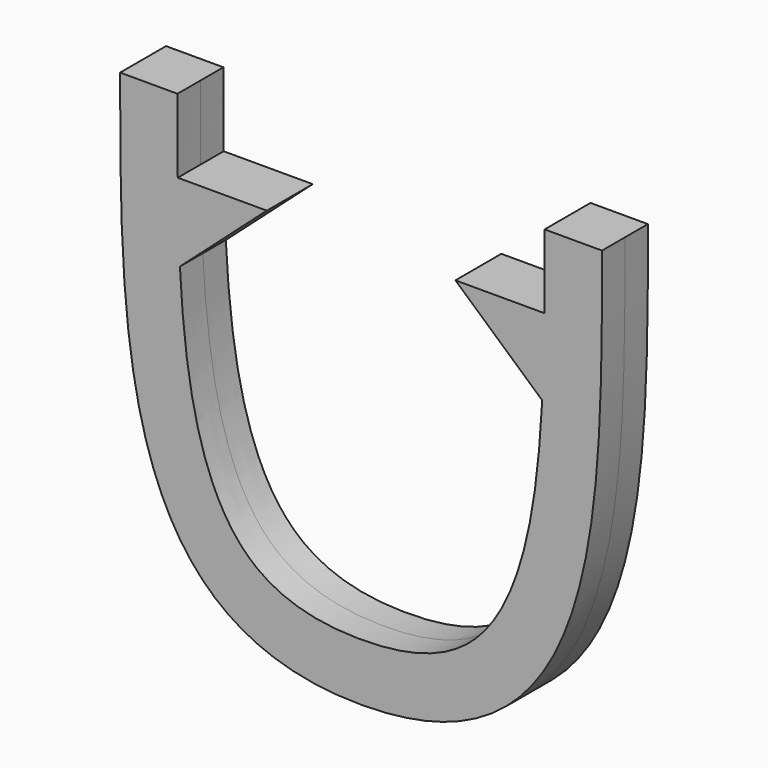
from build123d import *

# Parameters (mm, degrees)
F1_DEPTH = 5


# Not quite as in the source:
# - ends of sketch curves that miss each other by under 0.0002 mm in the source are joined
# - the dataset's text gives a spline's control points without its knots; the knots are read off the source's solid


with BuildPart() as f1:
    # F0 (on Front) → F1 (new body, symmetric)
    with BuildSketch(Plane.XZ):
        with BuildLine():
            add(Edge.make_bspline(
                [(0, 0), (-42, 0), (-42, 41.675), (-42, 83.35)],
                knots=[0, 0, 0, 0, 93.3339300576, 93.3339300576, 93.3339300576, 93.3339300576], degree=3))
            add(Edge.make_bspline(
                [(0, 0), (42, 0), (42, 41.675), (42, 83.35)],
                knots=[0, 0, 0, 0, 93.3339300576, 93.3339300576, 93.3339300576, 93.3339300576], degree=3))
            Line((42, 83.35), (32, 83.35))
            add(Edge.make_bspline(
                [(31.9530673006, 70.4800003254), (31.9996895611, 74.700760082), (32, 79.0074224925), (32, 83.35)],
                knots=[0.89579898, 0.89579898, 0.89579898, 0.89579898, 1, 1, 1, 1], degree=3))
            add(Edge.make_bspline(
                [(31.5750922391, 56.9799976128), (31.7546010541, 60.5369260512), (31.8825219764, 65.0296170648), (31.9437612931, 69.6375181896), (31.9530673006, 70.4800003254)],
                knots=[0.7815762928, 0.7815762928, 0.7815762928, 0.7815762928, 0.875, 0.89579898, 0.89579898, 0.89579898, 0.89579898], degree=3))
            add(Edge.make_bspline(
                [(0, 10), (2.2115575397, 10), (6.2274929739, 10.2749181924), (11.1177347786, 11.3540494511), (15.0427811386, 12.9515249487), (18.2502684866, 14.996645723), (20.9855911418, 17.5385737315), (23.3948464447, 20.6936265453), (25.5136174291, 24.5488626614), (27.3249436294, 29.1192747786), (28.8101204922, 34.361966709), (30.3563502536, 42.1519217161), (31.1711492212, 49.8831114238), (31.5144200278, 55.777790839), (31.5750922391, 56.9799976128)],
                knots=[0, 0, 0, 0, 0.0625, 0.125, 0.1875, 0.25, 0.3125, 0.375, 0.4375, 0.5, 0.5625, 0.625, 0.75, 0.7815762928, 0.7815762928, 0.7815762928, 0.7815762928], degree=3))
            add(Edge.make_bspline(
                [(0, 10), (-2.2115575397, 10), (-6.2274929739, 10.2749181924), (-11.1177347786, 11.3540494511), (-15.0427811386, 12.9515249487), (-18.2502684866, 14.996645723), (-20.9855911418, 17.5385737315), (-23.3948464447, 20.6936265453), (-25.5136174291, 24.5488626614), (-27.3249436294, 29.1192747786), (-28.8101204922, 34.361966709), (-30.3563502536, 42.1519217161), (-31.1711492212, 49.8831114238), (-31.5144200278, 55.777790839), (-31.5750922391, 56.9799976128)],
                knots=[0, 0, 0, 0, 0.0625, 0.125, 0.1875, 0.25, 0.3125, 0.375, 0.4375, 0.5, 0.5625, 0.625, 0.75, 0.7815762928, 0.7815762928, 0.7815762928, 0.7815762928], degree=3))
            add(Edge.make_bspline(
                [(-31.5750922391, 56.9799976128), (-31.7546010541, 60.5369260512), (-31.8825219764, 65.0296170648), (-31.9437612931, 69.6375181896), (-31.9530673006, 70.4800003254)],
                knots=[0.7815762928, 0.7815762928, 0.7815762928, 0.7815762928, 0.875, 0.89579898, 0.89579898, 0.89579898, 0.89579898], degree=3))
            add(Edge.make_bspline(
                [(-31.9530673006, 70.4800003254), (-31.9996895611, 74.700760082), (-32, 79.0074224925), (-32, 83.35)],
                knots=[0.89579898, 0.89579898, 0.89579898, 0.89579898, 1, 1, 1, 1], degree=3))
            Line((-32, 83.35), (-42, 83.35))
        make_face()
        with BuildLine():
            add(Edge.make_bspline(
                [(31.5750922391, 56.9799976128), (31.7546010541, 60.5369260512), (31.8825219764, 65.0296170648), (31.9437612931, 69.6375181896), (31.9530673006, 70.4800003254)],
                knots=[0.7815762928, 0.7815762928, 0.7815762928, 0.7815762928, 0.875, 0.89579898, 0.89579898, 0.89579898, 0.89579898], degree=3))
            Line((31.9530673006, 70.4800003254), (16.4530926609, 70.4800000453))
            Line((16.4530926609, 70.4800000453), (31.5750922391, 56.9799976128))
        make_face()
        with BuildLine():
            Line((-16.4265166968, 70.4800000453), (-31.9530926609, 70.4800000453))
            add(Edge.make_bspline(
                [(-31.5750922391, 56.9799976128), (-31.7546010541, 60.5369260512), (-31.8825219764, 65.0296170648), (-31.9437612931, 69.6375181896), (-31.9530926609, 70.4800000453)],
                knots=[0.7815762928, 0.7815762928, 0.7815762928, 0.7815762928, 0.875, 0.89579898, 0.89579898, 0.89579898, 0.89579898], degree=3))
            Line((-31.5750922391, 56.9799976128), (-16.4265166968, 70.4800000453))
        make_face()
    extrude(amount=F1_DEPTH, both=True)


solid = f1.part
